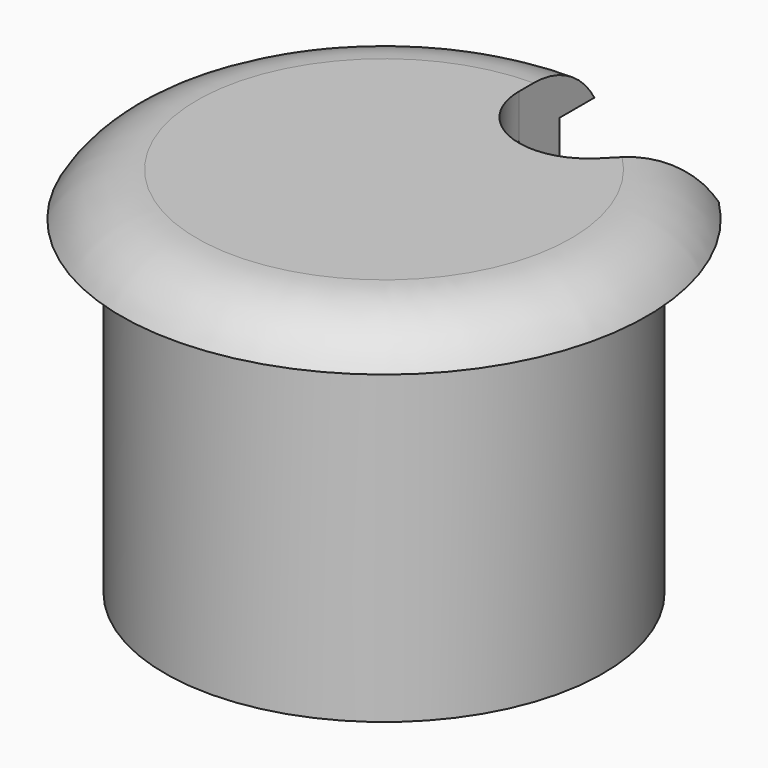
from build123d import *

# Parameters (mm, degrees)
F1_ANGLE    = 315
F2_T2_ANGLE = 359.64
F4_DEPTH    = 2.54


# Not quite as in the source:
# - a fillet or chamfer that OpenCascade refuses, or shapes differently, is made with other operations: its cross-section is extruded or revolved along the edge and cut away or added


with BuildPart() as f1:
    # F0 (on Right) → F1 (revolve)
    with BuildSketch(Plane.YZ):
        Polygon((15.24, 21.59), (0, 21.59), (0, 19.05), (9.7782645518, 19.05), (9.7782645518, 0), (12.7, 0), (12.7, 19.05), (15.24, 19.05), align=None)
    revolve(axis=Axis((0, 0, 20.32), (0, 0, 1)), revolution_arc=F1_ANGLE)

    # F2: fillet of radius 5.08 on 1 edges, made by hand

    # F2_s1 → F2_t2 (revolve, cut)
    with BuildSketch(Plane(origin=(0, 0, 0), x_dir=(0, 0, 1), z_dir=(0.9250772068, -0.3797790955, 0))):
        with BuildLine():
            ThreePointArc((21.59, -10.8405909488), (20.9094090512, -13.3805909488), (19.05, -15.24))
            Line((19.05, -15.24), (21.59, -15.24))
            Line((21.59, -15.24), (21.59, -10.8405909488))
        make_face()
    revolve(axis=Axis((0, 0, 21.59), (0, 0, 1)), revolution_arc=F2_T2_ANGLE, mode=Mode.SUBTRACT)

    # F3 (on face) → F4 (join)
    with BuildSketch(Plane(origin=(0, 0, 19.05), x_dir=(1, 0, 0), z_dir=(0, 0, -1))):
        with BuildLine():
            ThreePointArc((0, -9.7782645518), (2.5003109935, -6.0362847106), (6.9142771728, -6.9142771728))
            Line((6.9142771728, -6.9142771728), (0, 0))
            Line((0, 0), (0, -9.7782645518))
        make_face()
    extrude(amount=-F4_DEPTH)


solid = f1.part
